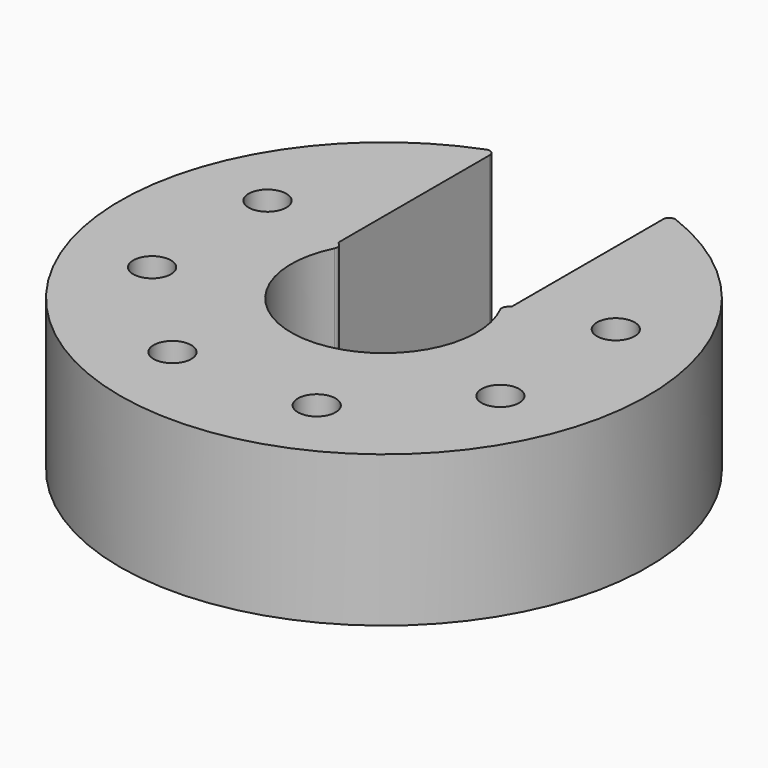
from build123d import *

# Parameters (mm, degrees)
F3_DEPTH = 12.7
F4_R     = 0.508
F2_R     = 1.5875
F5_DEPTH = 12.7


# Not quite as in the source:
# - a variable given as a bare number and used for a length is read in inches; the dataset says mm whatever the document's units were


with BuildPart() as f3:
    # F1 (on Top) → F3 (new body)
    with BuildSketch(Plane.XY):
        with BuildLine():
            Line((-7.3025, 4.3464899063), (-7.3025, 20.9910485386))
            ThreePointArc((-7.3025, 20.9910485386), (0, -22.225), (7.3025, 20.9910485386))
            Line((7.3025, 20.9910485386), (7.3025, 4.3464899063))
            Line((7.3025, 4.3464899063), (6.7952360256, 3.8508022029))
            ThreePointArc((6.7952360256, 3.8508022029), (0, -7.8105), (-6.7952360256, 3.8508022029))
            Line((-6.7952360256, 3.8508022029), (-7.3025, 4.3464899063))
        make_face()
    extrude(amount=F3_DEPTH)

    # F4
    f4_edges = [f3.edges().sort_by_distance(p)[0] for p in [
        (-6.795236, 3.850802, 6.35),
        (6.795236, 3.850802, 6.35),
        (-7.3025, 20.991049, 6.35),
        (7.3025, 20.991049, 6.35),
    ]]
    fillet(f4_edges, radius=F4_R)

    # F2 (on Top) → F5 (cut, through all)
    with BuildSketch(Plane.XY):
        with Locations((-14.6665875786, 6.0750994888)):
            Circle(F2_R)
        with Locations((-14.6665875786, -6.0750994888)):
            Circle(F2_R)
        with Locations((-6.0750994888, -14.6665875786)):
            Circle(F2_R)
        with Locations((6.0750994888, -14.6665875786)):
            Circle(F2_R)
        with Locations((14.6665875786, -6.0750994888)):
            Circle(F2_R)
        with Locations((14.6665875786, 6.0750994888)):
            Circle(F2_R)
    extrude(amount=F5_DEPTH, mode=Mode.SUBTRACT)


solid = f3.part
